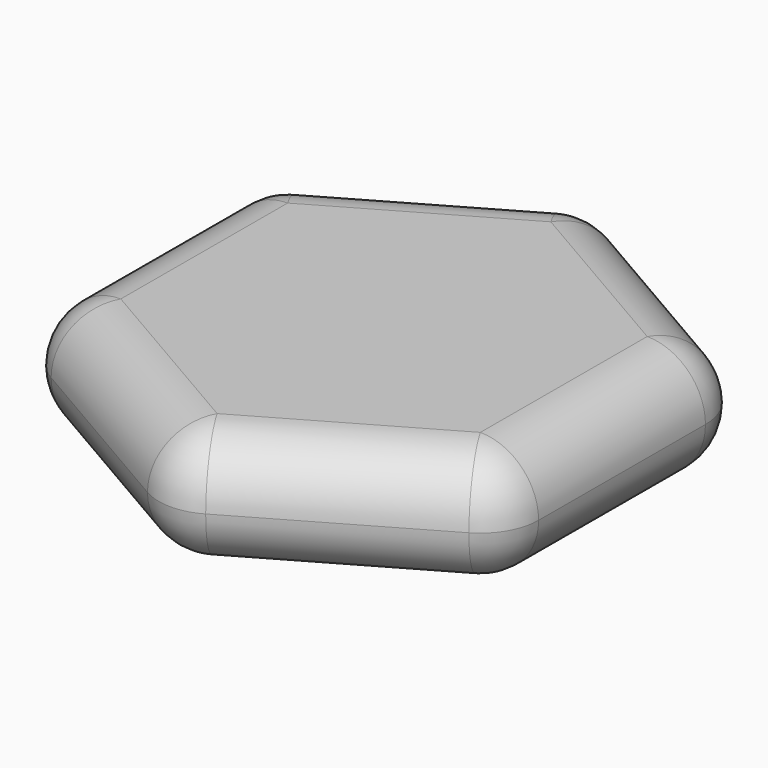
from build123d import *

# Parameters (mm, degrees)
F1_DEPTH = 25.4
F2_R     = 12.69999


# Not quite as in the source:
# - a fillet or chamfer is up to 0.001 mm smaller than in the source, because OpenCascade refuses the exact size


with BuildPart() as f1:
    # F0 (on Top) → F1 (new body)
    with BuildSketch(Plane.XY):
        Polygon((51.9719609901, 29.8469270905), (0.1377834097, 59.9325020472), (-51.8341775803, 30.0855749566), (-51.9719609901, -29.8469270905), (-0.1377834097, -59.9325020472), (51.8341775803, -30.0855749566), align=None)
    extrude(amount=F1_DEPTH)

    # F2 (radius 12.7 in the source; OpenCascade refuses exactly that, so slightly less here)
    f2_edges = [f1.edges().sort_by_distance(p)[0] for p in [
        (51.971961, 29.846927, 12.7),
        (0.137783, 59.932502, 12.7),
        (26.054872, 44.889715, 0),
        (26.054872, 44.889715, 25.4),
        (-51.834178, 30.085575, 12.7),
        (-25.848197, 45.009039, 0),
        (-25.848197, 45.009039, 25.4),
        (-51.971961, -29.846927, 12.7),
        (-51.903069, 0.119324, 0),
        (-51.903069, 0.119324, 25.4),
        (-0.137783, -59.932502, 12.7),
        (51.834178, -30.085575, 12.7),
        (25.848197, -45.009039, 0),
        (25.848197, -45.009039, 25.4),
        (-26.054872, -44.889715, 0),
        (-26.054872, -44.889715, 25.4),
        (51.903069, -0.119324, 0),
        (51.903069, -0.119324, 25.4),
    ]]
    fillet(f2_edges, radius=F2_R)


solid = f1.part
